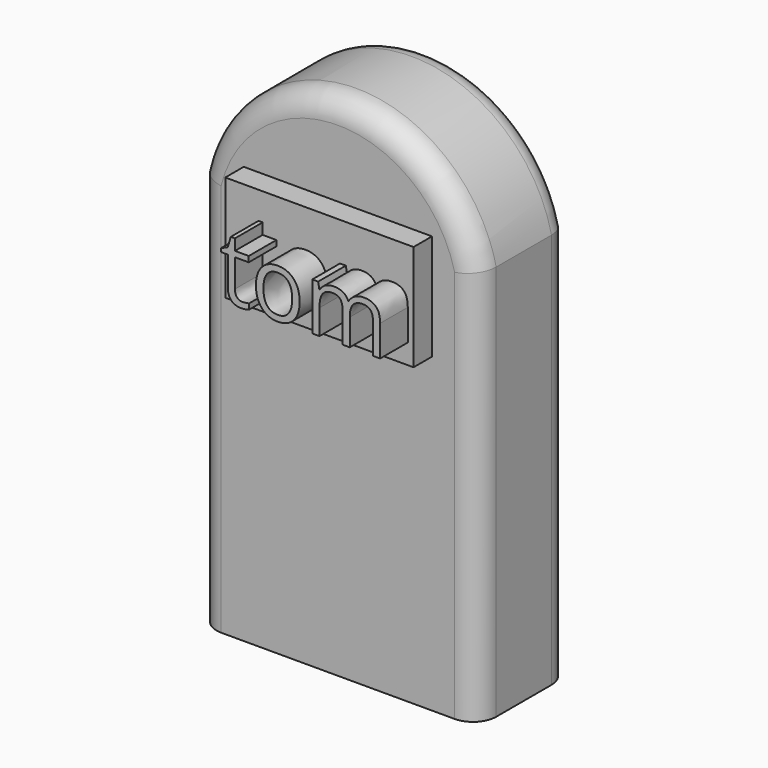
from build123d import *

# Parameters (mm, degrees)
F0_W         = 61.5904293954
F0_H         = 87.2051473707
F0_W_2       = 33.9610800147
F0_H_2       = 7.4328972495
F1_DEPTH     = 25.4
F2_T1_DEPTH  = 112.6051473707
F2_T4_ANGLE  = 200.7857698038
F2_T6_ANGLE  = 200.7857698038
F3_W         = 41.457798332
F3_H         = 23.3177287972
F4_DEPTH     = 5.08
F5_TEXT_SIZE = 19.5697622581
F6_DEPTH     = 7.62


# Not quite as in the source:
# - a fillet or chamfer that OpenCascade refuses, or shapes differently, is made with other operations: its cross-section is extruded or revolved along the edge and cut away or added
# - Text() gives the source's letters only with a copy of the font that has no kerning and outlines rounded to 1/6400 em; it was checked with that copy


with BuildPart() as f1:
    # F0 (on Front) → F1 (new body)
    with BuildSketch(Plane.XZ):
        with BuildLine():
            ThreePointArc((25.9025171399, 29.0683824569), (-4.8926975578, 53.7018686048), (-35.6879122555, 29.0683824569))
            Line((-35.6879122555, 29.0683824569), (25.9025171399, 29.0683824569))
        make_face()
        with Locations((-4.8926975578, -14.5341912284)):
            Rectangle(F0_W, F0_H)
        with Locations((-4.8926975578, 22.136017983)):
            Rectangle(F0_W_2, F0_H_2, mode=Mode.SUBTRACT)
        with Locations((-4.8926975578, 22.136017983)):
            Rectangle(F0_W_2, F0_H_2)
    extrude(amount=F1_DEPTH)

    # F2: fillet of radius 5.08 on 6 edges, made by hand

    # F2_s2 → F2_t1 (cut)
    with BuildSketch(Plane.XY.offset(-70.8367649138)):
        with BuildLine():
            ThreePointArc((-35.6879122555, -20.32), (-34.200014704, -23.9121024484), (-30.6079122555, -25.4))
            Line((-30.6079122555, -25.4), (-35.6879122555, -25.4))
            Line((-35.6879122555, -25.4), (-35.6879122555, -20.32))
        make_face()
        with BuildLine():
            ThreePointArc((25.9025171399, -20.32), (24.4146195883, -23.9121024484), (20.8225171399, -25.4))
            Line((20.8225171399, -25.4), (25.9025171399, -25.4))
            Line((25.9025171399, -25.4), (25.9025171399, -20.32))
        make_face()
        with BuildLine():
            ThreePointArc((25.9025171399, -5.08), (24.4146195883, -1.4878975516), (20.8225171399, 0))
            Line((20.8225171399, 0), (25.9025171399, 0))
            Line((25.9025171399, 0), (25.9025171399, -5.08))
        make_face()
        with BuildLine():
            ThreePointArc((-35.6879122555, -5.08), (-34.200014704, -1.4878975516), (-30.6079122555, 0))
            Line((-30.6079122555, 0), (-35.6879122555, 0))
            Line((-35.6879122555, 0), (-35.6879122555, -5.08))
        make_face()
    extrude(amount=F2_T1_DEPTH, mode=Mode.SUBTRACT)

    # F2_s3 → F2_t4 (revolve, cut)
    with BuildSketch(Plane(origin=(3.7685337563, 0, 20.5474963435), x_dir=(0, 1, 0), z_dir=(-0.1803970021, 0, -0.9835938804))):
        with BuildLine():
            ThreePointArc((-5.08, 22.7601519626), (-1.4878975516, 21.2722544111), (0, 17.6801519626))
            Line((0, 17.6801519626), (0, 22.7601519626))
            Line((0, 22.7601519626), (-5.08, 22.7601519626))
        make_face()
    revolve(axis=Axis((-4.8926975578, 0, 22.136017983), (0, -1, 0)), revolution_arc=F2_T4_ANGLE, mode=Mode.SUBTRACT)

    # F2_s5 → F2_t6 (revolve, cut)
    with BuildSketch(Plane(origin=(3.7685337563, 0, 20.5474963435), x_dir=(0, 1, 0), z_dir=(-0.1803970021, 0, -0.9835938804))):
        with BuildLine():
            ThreePointArc((-20.32, 22.7601519626), (-23.9121024484, 21.2722544111), (-25.4, 17.6801519626))
            Line((-25.4, 17.6801519626), (-25.4, 22.7601519626))
            Line((-25.4, 22.7601519626), (-20.32, 22.7601519626))
        make_face()
    revolve(axis=Axis((-4.8926975578, -25.4, 22.136017983), (0, -1, 0)), revolution_arc=F2_T6_ANGLE, mode=Mode.SUBTRACT)

    # F3 (on face) → F4 (join)
    with BuildSketch(Plane.XZ.offset(25.4)):
        with Locations((-4.8926975578, 22.136017983)):
            Rectangle(F3_W, F3_H)
    extrude(amount=F4_DEPTH)

    # F5 (on face) → F6 (join)
    with BuildSketch(Plane.XZ.offset(30.48)):
        with Locations((-20.7776004665, 14.8624926805)):
            Text('tom', F5_TEXT_SIZE, font='Open Sans', text_align=(TextAlign.LEFT, TextAlign.BOTTOM))
    extrude(amount=F6_DEPTH)


solid = f1.part
